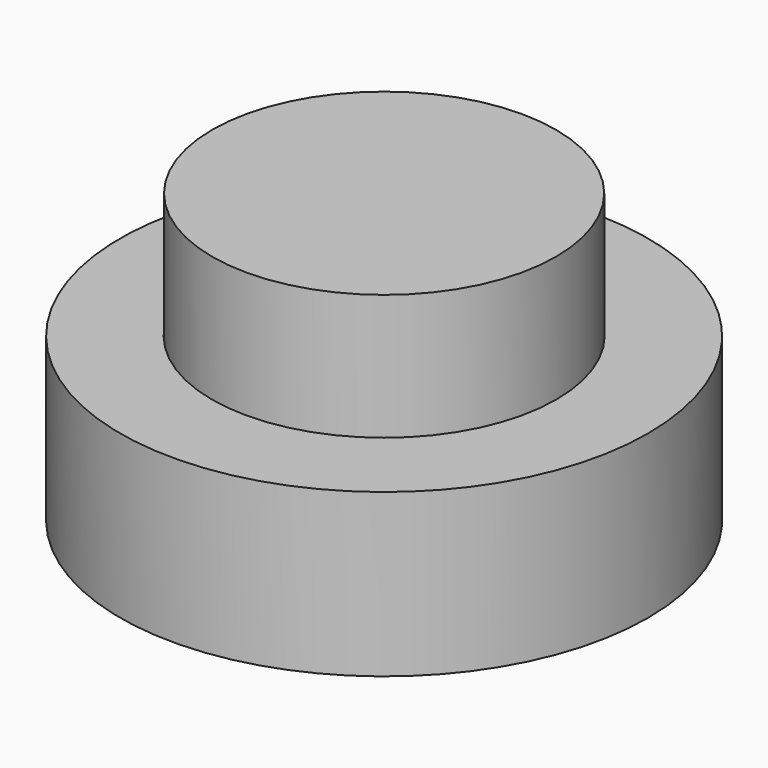
from build123d import *

# Parameters (mm, degrees)
F3_R     = 77.8669465494
F4_DEPTH = 47.8855650872
F5_D     = 101.6
F8_R     = 50.7080101121
F9_DEPTH = 84.9374663085


# Not quite as in the source:
# - the program builds the solid bodies; features that only make, move or delete a surface that nothing else refers to are left out


with BuildPart() as f4:
    # F3 (on face) → F4 (new body)
    with BuildSketch(Plane.XY):
        Circle(F3_R)
    extrude(amount=F4_DEPTH)

    # F5 (through all)
    with Locations(Plane(origin=(0, 0, 0), x_dir=(1, 0, 0), z_dir=(0, 0, -1))):
        with Locations((0, 0)):
            Hole(F5_D / 2)


with BuildPart() as f9:
    # F8 (on face) → F9 (new body)
    with BuildSketch(Plane.XY):
        Circle(F8_R)
    extrude(amount=F9_DEPTH)


solid = Compound([f4.part, f9.part])
